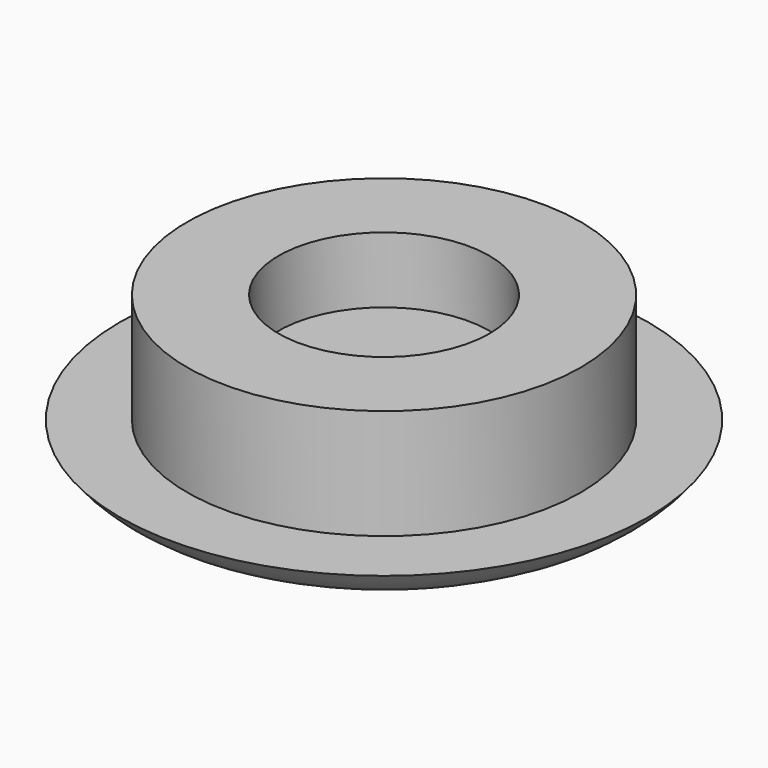
from build123d import *

# Parameters (mm, degrees)
F0_R     = 12
F1_DEPTH = 2
F2_R     = 8.9467567694
F3_DEPTH = 5
F4_R     = 4.7902731663
F5_DEPTH = 3


# Not quite as in the source:
# - a fillet or chamfer that OpenCascade refuses, or shapes differently, is made with other operations: its cross-section is extruded or revolved along the edge and cut away or added


with BuildPart() as f1:
    # F0 (on Top) → F1 (new body)
    with BuildSketch(Plane.XY):
        Circle(F0_R)
    extrude(amount=F1_DEPTH)

    # F2 (on face) → F3 (join)
    with BuildSketch(Plane.XY.offset(2)):
        Circle(F2_R)
    extrude(amount=F3_DEPTH)

    # F4 (on face) → F5 (cut)
    with BuildSketch(Plane.XY.offset(7)):
        Circle(F4_R)
    extrude(amount=-F5_DEPTH, mode=Mode.SUBTRACT)

    # F6: fillet of radius 5 on 1 edges, made by hand

    # F6_s1 → F6_t2 (revolve, cut)
    with BuildSketch(Plane.XZ):
        with BuildLine():
            ThreePointArc((12, 2), (10.2360679775, 0.527864045), (8, 0))
            Line((8, 0), (12, 0))
            Line((12, 0), (12, 2))
        make_face()
    revolve(axis=Axis((0, 0, 0), (0, 0, 1)), mode=Mode.SUBTRACT)


solid = f1.part
